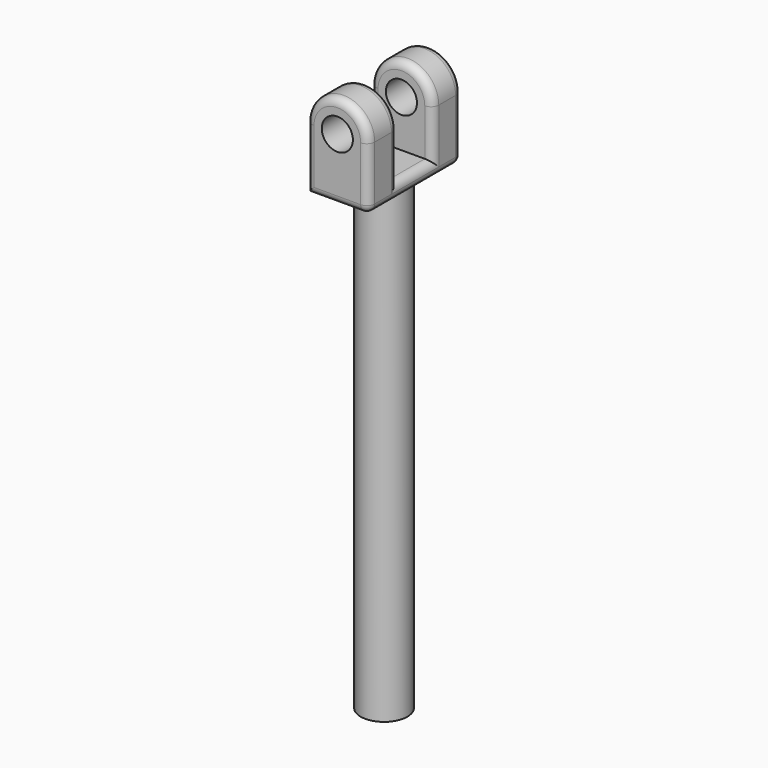
from build123d import *

# Parameters (mm, degrees)
F0_R          = 5
F1_DEPTH      = 18.75
F1_DEPTH_BACK = 18.75
F4_DEPTH      = 7
F4_DEPTH_BACK = 7
F6_R          = 7.5
F7_DEPTH      = 150
F8_R          = 2.49999


# Not quite as in the source:
# - a fillet or chamfer is up to 0.001 mm smaller than in the source, because OpenCascade refuses the exact size
# - a feature names something its author has since deleted; it is built from what else it names


with BuildPart() as f1:
    # F0 (on Front) → F1 (new body, two sides)
    with BuildSketch(Plane.XZ) as f1_sk:
        with BuildLine():
            Line((10, 0), (10, 20))
            ThreePointArc((10, 20), (0, 30), (-10, 20))
            Line((-10, 20), (-10, 0))
            Line((-10, 0), (10, 0))
        make_face()
        with Locations((0, 20)):
            Circle(F0_R, mode=Mode.SUBTRACT)
    extrude(amount=F1_DEPTH)
    extrude(f1_sk.sketch, amount=-F1_DEPTH_BACK)

    # F3 (on offset) → F4 (cut, two sides)
    with BuildSketch(Plane.XZ) as f4_sk:
        Polygon((-12, 5), (0, 5), (12, 5), (12, 35), (-12, 35), align=None)
    extrude(amount=-F4_DEPTH, mode=Mode.SUBTRACT)
    extrude(f4_sk.sketch, amount=F4_DEPTH_BACK, mode=Mode.SUBTRACT)

    # F6 (on offset) → F7 (join)
    with BuildSketch(Plane(origin=(0, 0, 0), x_dir=(1, 0, 0), z_dir=(0, 0, -1))):
        Circle(F6_R)
    extrude(amount=F7_DEPTH)

    # F8 (radius 2.5 in the source; OpenCascade refuses exactly that, so slightly less here)
    f8_edges = [f1.edges().sort_by_distance(p)[0] for p in [
        (10, -7, 12.5),
        (10, 7, 12.5),
        (10, 18.75, 10),
        (10, -18.75, 10),
        (10, 0, 5),
        (-10, 0, 5),
        (10, 0, 0),
        (0, 18.75, 0),
        (0, -18.75, 0),
    ]]
    fillet(f8_edges, radius=F8_R)


solid = f1.part
